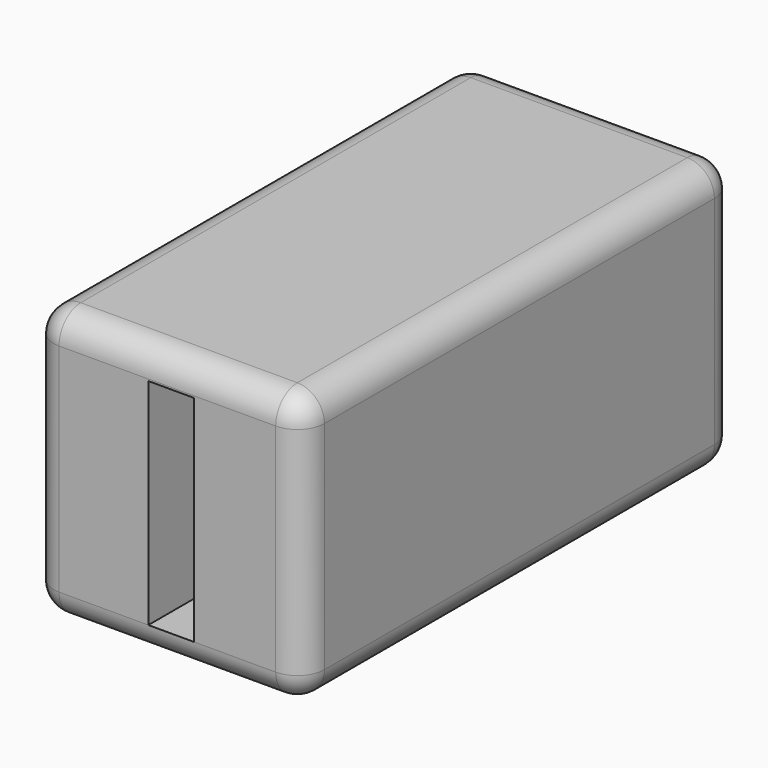
from build123d import *

# Parameters (mm, degrees)
F0_W         = 10
F0_H         = 10
F1_DEPTH     = 20
F2_R         = 1
F3_TEXT_SIZE = 11.1111111111
F4_DEPTH     = 20


# Not quite as in the source:
# - Text() gives the source's letters only with a copy of the font that has no kerning and outlines rounded to 1/6400 em; it was checked with that copy


with BuildPart() as f1:
    # F0 (on Front) → F1 (new body)
    with BuildSketch(Plane.XZ):
        with Locations((5, 5)):
            Rectangle(F0_W, F0_H)
    extrude(amount=F1_DEPTH)

    # F2
    f2_edges = [f1.edges().sort_by_distance(p)[0] for p in [
        (10, -10, 10),
        (0, -10, 10),
        (5, 0, 10),
        (5, -20, 10),
        (10, -10, 0),
        (10, 0, 5),
        (10, -20, 5),
        (0, -10, 0),
        (5, 0, 0),
        (5, -20, 0),
        (0, 0, 5),
        (0, -20, 5),
    ]]
    fillet(f2_edges, radius=F2_R)

    # F3 (on face) → F4 (cut)
    with BuildSketch(Plane.XZ.offset(20)):
        with Locations((3.2994791667, 1)):
            Text('I', F3_TEXT_SIZE, font='Open Sans', font_style=FontStyle.BOLD, text_align=(TextAlign.LEFT, TextAlign.BOTTOM))
    extrude(amount=-F4_DEPTH, mode=Mode.SUBTRACT)


solid = f1.part
